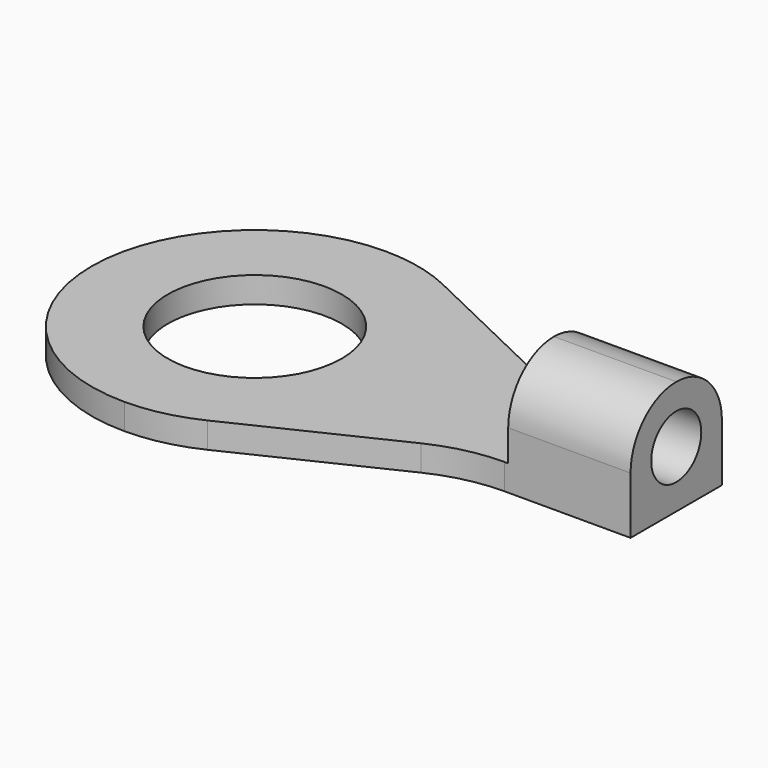
from build123d import *

# Parameters (mm, degrees)
F0_R     = 3.2
F1_DEPTH = 0.95
F2_W     = 4.5
F2_H     = 4.2
F3_DEPTH = 3.25
F4_R     = 2.09999
F5_R     = 1.15
F6_DEPTH = 25


# Not quite as in the source:
# - a fillet or chamfer is up to 0.001 mm smaller than in the source, because OpenCascade refuses the exact size


with BuildPart() as f1:
    # F0 (on Top) → F1 (new body)
    with BuildSketch(Plane.XY):
        with BuildLine():
            Line((16.8637172922, 3.9), (21.5, 3.9))
            Line((21.5, 3.9), (21.5, 8.1))
            Line((21.5, 8.1), (16.8637172922, 8.1))
            ThreePointArc((16.8637172922, 8.1), (15.5339156309, 8.2492199202), (14.2702582689, 8.6894574861))
            Line((14.2702582689, 8.6894574861), (8.5934590232, 11.4105425139))
            ThreePointArc((8.5934590232, 11.4105425139), (7.3298016613, 11.8507800798), (6, 12))
            ThreePointArc((6, 12), (1.7573593129, 10.2426406871), (0, 6))
            ThreePointArc((0, 6), (1.7573593129, 1.7573593129), (6, 0))
            ThreePointArc((6, 0), (7.3298016613, 0.1492199202), (8.5934590232, 0.5894574861))
            Line((8.5934590232, 0.5894574861), (14.2702582689, 3.3105425139))
            ThreePointArc((14.2702582689, 3.3105425139), (15.5339156309, 3.7507800798), (16.8637172922, 3.9))
        make_face()
        with Locations((6, 6)):
            Circle(F0_R, mode=Mode.SUBTRACT)
    extrude(amount=F1_DEPTH)

    # F2 (on face) → F3 (join)
    with BuildSketch(Plane.XY.offset(0.95)):
        with Locations((19.25, 6)):
            Rectangle(F2_W, F2_H)
    extrude(amount=F3_DEPTH)

    # F4 (radius 2.1 in the source; OpenCascade refuses exactly that, so slightly less here)
    f4_edges = [f1.edges().sort_by_distance(p)[0] for p in [
        (19.25, 8.1, 4.2),
        (19.25, 3.9, 4.2),
    ]]
    fillet(f4_edges, radius=F4_R)

    # F5 (on face) → F6 (cut)
    with BuildSketch(Plane.YZ.offset(21.5)):
        with Locations((6, 2.1)):
            Circle(F5_R)
    extrude(amount=-F6_DEPTH, mode=Mode.SUBTRACT)


solid = f1.part
